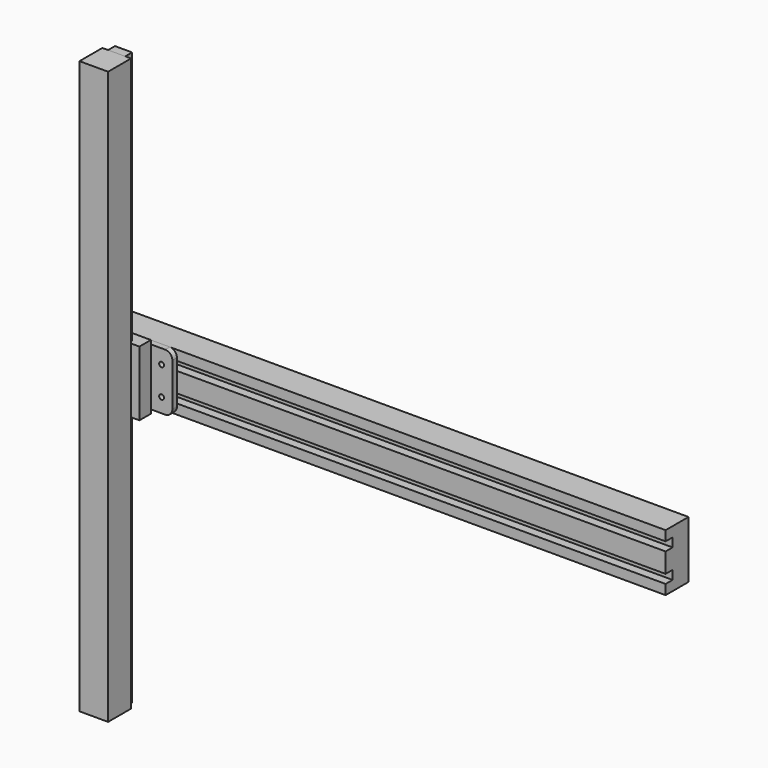
from build123d import *

# Parameters (mm, degrees)
F0_W            = 400
F0_H            = 40
F1_DEPTH        = 20
F2_W            = 400
F2_H            = 6.2
F3_DEPTH        = 6.1
F5_W            = 27
F5_H            = 45.4
F6_DEPTH        = 10
F7_D            = 2.5
F7_DEPTH        = 6
F7_TIP          = 0.7510757738
F8_W            = 15
F8_H            = 40
F8_W_2          = 27
F8_R            = 1.25
F9_DEPTH        = 4
F11_D           = 3.4
F11_CSINK_D     = 6.72
F11_CSINK_ANGLE = 90
F12_D           = 3.4
F13_R           = 5
F14_W           = 12
F14_H           = 3
F15_DEPTH       = 177.3
F15_DEPTH_BACK  = 222.7
F16_W           = 20
F16_H           = 400
F17_DEPTH       = 20


with BuildPart() as f1:
    # F0 (on Front) → F1 (new body)
    with BuildSketch(Plane.XZ):
        Rectangle(F0_W, F0_H)
    extrude(amount=-F1_DEPTH)

    # F2 (on face) → F3 (cut)
    with BuildSketch(Plane.XZ):
        with Locations((0, 10)):
            Rectangle(F2_W, F2_H)
        with Locations((0, -10)):
            Rectangle(F2_W, F2_H)
    extrude(amount=-F3_DEPTH, mode=Mode.SUBTRACT)


with BuildPart() as f6:
    # F5 (on offset) → F6 (new body)
    with BuildSketch(Plane.XZ.offset(4)):
        with Locations((-170, 0)):
            Rectangle(F5_W, F5_H)
    extrude(amount=F6_DEPTH)

    # F7
    with Locations(Plane(origin=(0, -4, 0), x_dir=(1, 0, 0), z_dir=(0, 1, 0))):
        with Locations((-160, -10), (-180, -10), (-160, 10), (-180, 10)):
            Hole(F7_D / 2, depth=F7_DEPTH)
            with Locations((0, 0, -(F7_DEPTH + F7_TIP / 2))):  # 118° drill point
                Cone(0, F7_D / 2, F7_TIP, mode=Mode.SUBTRACT)

    # F14 (on face) → F15 (join, two sides)
    with BuildSketch(Plane.XY.offset(22.7)) as f15_sk:
        with Locations((-170, -15.5)):
            Rectangle(F14_W, F14_H)
        with Locations((-170, -12.5)):
            Rectangle(F14_W, F14_H)
    extrude(amount=F15_DEPTH)
    extrude(f15_sk.sketch, amount=-F15_DEPTH_BACK)


with BuildPart() as f9:
    # F8 (on face) → F9 (new body)
    with BuildSketch(Plane(origin=(0, -4, 0), x_dir=(-1, 0, 0), z_dir=(0, 1, 0))):
        with Locations((191, 0)):
            Rectangle(F8_W, F8_H)
        with Locations((170, 0)):
            Rectangle(F8_W_2, F8_H)
        with Locations((160, -10)):
            Circle(F8_R, mode=Mode.SUBTRACT)
        with Locations((180, -10)):
            Circle(F8_R, mode=Mode.SUBTRACT)
        with Locations((160, 10)):
            Circle(F8_R, mode=Mode.SUBTRACT)
        with Locations((180, 10)):
            Circle(F8_R, mode=Mode.SUBTRACT)
        with Locations((149, 0)):
            Rectangle(F8_W, F8_H)
    extrude(amount=F9_DEPTH)

    # F11 (through all)
    with Locations(Plane(origin=(0, 0, 0), x_dir=(-1, 0, 0), z_dir=(0, 1, 0))):
        with Locations((160, 10), (180, 10), (160, -10), (180, -10)):
            CounterSinkHole(F11_D / 2, F11_CSINK_D / 2, counter_sink_angle=F11_CSINK_ANGLE)

    # F12 (through all)
    with Locations(Plane(origin=(0, -4, 0), x_dir=(-1, 0, 0), z_dir=(0, -1, 0))):
        with Locations((191, -10), (191, 10), (149, -10), (149, 10)):
            Hole(F12_D / 2)

    # F13
    f13_edges = [f9.edges().sort_by_distance(p)[0] for p in [
        (-198.5, -2, 20),
        (-141.5, -2, 20),
        (-198.5, -2, -20),
        (-141.5, -2, -20),
    ]]
    fillet(f13_edges, radius=F13_R)


with BuildPart() as f17:
    # F16 (on face) → F17 (new body)
    with BuildSketch(Plane.XZ.offset(17)):
        with Locations((-170, 0)):
            Rectangle(F16_W, F16_H)
    extrude(amount=F17_DEPTH)


solid = Compound([f1.part, f6.part, f9.part, f17.part])
